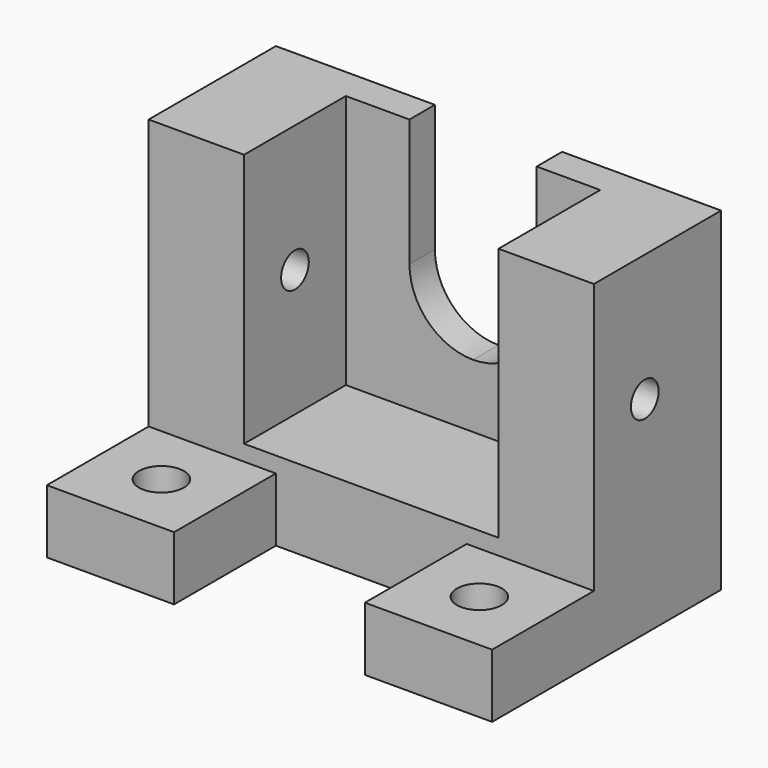
from build123d import *

# Parameters (mm, degrees)
F0_W     = 44.45
F0_H     = 33.3248
F1_DEPTH = 7.9375
F2_W     = 25.4
F2_H     = 25.4
F3_DEPTH = 12.7
F5_W     = 12.7
F5_H     = 19.05
F6_DEPTH = 3.176
F7_R     = 6.34999
F8_W     = 12.7
F8_H     = 6.35
F9_DEPTH = 12.7
F11_D    = 4.4958
F13_D    = 3.4544


# Not quite as in the source:
# - a fillet or chamfer is up to 0.001 mm smaller than in the source, because OpenCascade refuses the exact size
# - a pattern or mirror of a feature is missing from the dataset's text; its kind, count and spacing are read off the source's solid


with BuildPart() as f1:
    # F0 (on Front) → F1 (new body, symmetric)
    with BuildSketch(Plane.XZ):
        with Locations((0, 16.6624)):
            Rectangle(F0_W, F0_H)
    extrude(amount=F1_DEPTH, both=True)

    # F2 (on face) → F3 (cut)
    with BuildSketch(Plane.XZ.offset(7.9375)):
        with Locations((0, 20.6248)):
            Rectangle(F2_W, F2_H)
    extrude(amount=-F3_DEPTH, mode=Mode.SUBTRACT)

    # F5 (on face) → F6 (cut, through all)
    with BuildSketch(Plane.XZ.offset(-4.7625)):
        with Locations((0, 23.7998)):
            Rectangle(F5_W, F5_H)
    extrude(amount=-F6_DEPTH, mode=Mode.SUBTRACT)

    # F7 (radius 6.35 in the source; OpenCascade refuses exactly that, so slightly less here)
    f7_edges = [f1.edges().sort_by_distance(p)[0] for p in [
        (-6.35, 6.35, 14.2748),
        (6.35, 6.35, 14.2748),
    ]]
    fillet(f7_edges, radius=F7_R)

    # F8 (on face) → F9 (join)
    with BuildSketch(Plane(origin=(-22.225, 0, 0), x_dir=(0, -1, 0), z_dir=(-1, 0, 0))):
        with Locations((14.2875, 3.175)):
            Rectangle(F8_W, F8_H)
    f9 = extrude(amount=-F9_DEPTH)

    # F9_copies: F9 across plane
    add(f9.mirror(Plane(origin=(0, 0, 0), x_dir=(0, 0, 1), z_dir=(1, 0, 0))))

    # F11 (through all)
    with Locations(Plane.XY.offset(6.35)):
        with Locations((-15.875, -14.2875)):
            f11 = Hole(F11_D / 2)

    # F11_copies: F11 across plane
    add(f11.mirror(Plane(origin=(0, 0, 0), x_dir=(0, 0, 1), z_dir=(1, 0, 0))), mode=Mode.SUBTRACT)

    # F13 (through all)
    with Locations(Plane(origin=(-22.225, 0, 0), x_dir=(0, -1, 0), z_dir=(-1, 0, 0))):
        with Locations((1.5875, 20.6248)):
            Hole(F13_D / 2)


solid = f1.part
